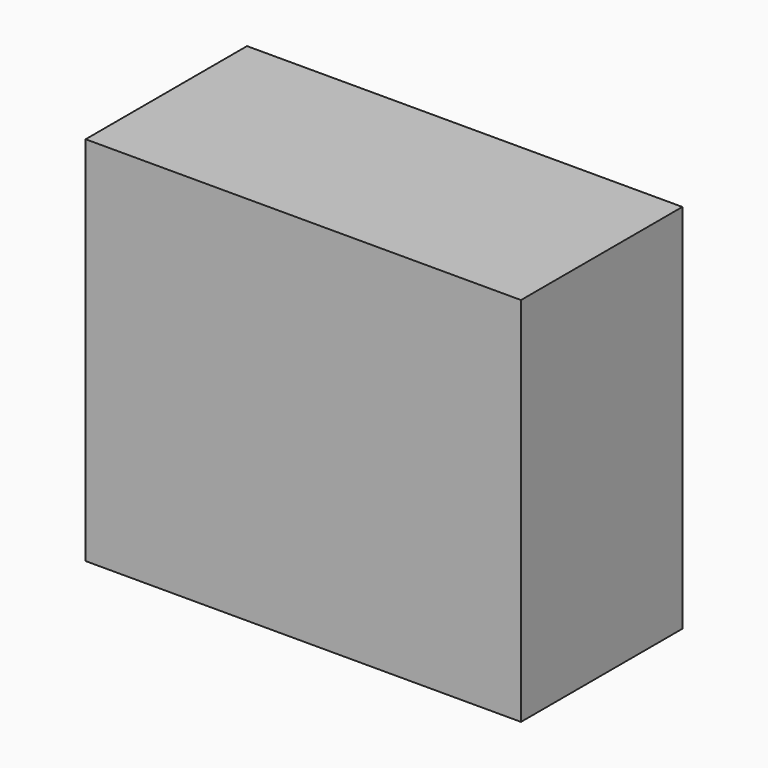
from build123d import *

# Parameters (mm, degrees)
F1_W     = 112.254448235
F1_H     = 52.0150326192
F2_DEPTH = 95.758
F0_W     = 112.254448235
F0_H     = 52.0150326192


with BuildPart() as f2:
    # F1 (on face) → F2 (new body)
    with BuildSketch(Plane.XY):
        with Locations((-6.6494457424, -26.0075163096)):
            Rectangle(F1_W, F1_H)
    extrude(amount=F2_DEPTH)


with BuildPart() as f2b:
    # F0 (on Top) → F2, piece 2 (new body)
    with BuildSketch(Plane.XY):
        with Locations((-6.6494457424, -26.0075163096)):
            Rectangle(F0_W, F0_H)
    extrude(amount=F2_DEPTH)


solid = Compound([f2.part, f2b.part])
